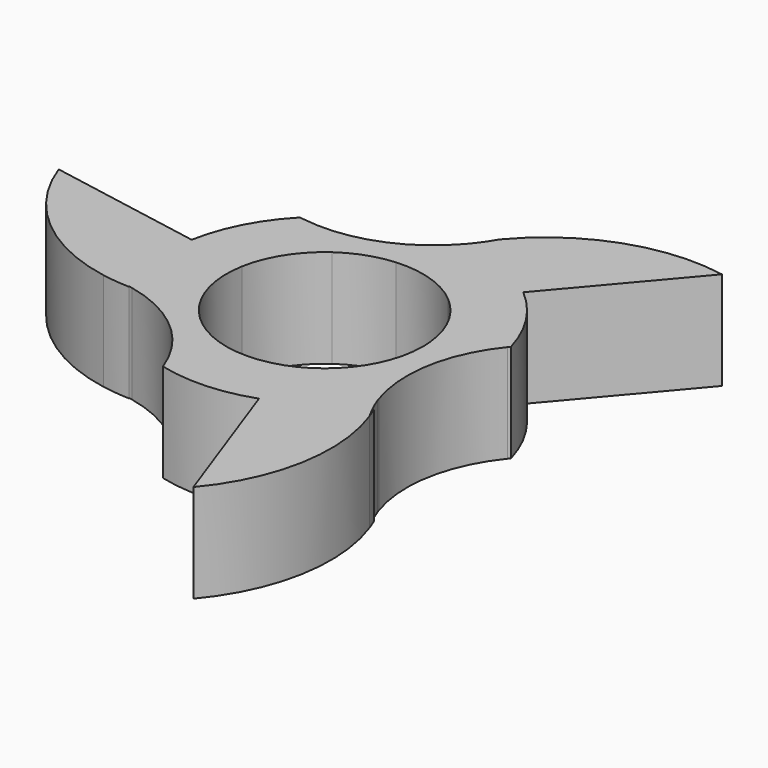
from build123d import *

# Parameters (mm, degrees)
F1_DEPTH = 12.7


# Not quite as in the source:
# - a feature of the source that left no trace in its solid (it failed there, or was rolled back) is left out


with BuildPart() as f1:
    # F0 (on Top) → F1 (new body)
    with BuildSketch(Plane.XY):
        with BuildLine():
            ThreePointArc((-7.3489403011, 10.3577544116), (-4.2883836636, 11.9540689957), (-0.9110245856, 12.667282037))
            ThreePointArc((-0.9110245856, 12.667282037), (0.2194109686, 16.5124994793), (1.9846889119, 20.1107456498))
            ThreePointArc((1.9846889119, 20.1107456498), (-5.3432740228, 15.0903277504), (-14.1828590922, 14.2154720724))
            ThreePointArc((-14.1828590922, 14.2154720724), (-10.6043004202, 12.5728851855), (-7.3489403011, 10.3577544116))
        make_face()
        with BuildLine():
            ThreePointArc((-18.6815829969, -8.250401529), (-18.454845536, -8.2932697378), (-18.2286800533, -8.3390598448))
            ThreePointArc((-18.2286800533, -8.3390598448), (-14.3209728725, -8.0523772846), (-10.5146757481, -7.1226114531))
            ThreePointArc((-10.5146757481, -7.1226114531), (-12.4259555067, -2.6240483505), (-12.4967192607, 2.263185304))
            Line((-12.4967192607, 2.263185304), (-20.0954213497, 3.6393281571))
            ThreePointArc((-20.0954213497, 3.6393281571), (-20.2794337822, -2.4114796562), (-18.6815829969, -8.250401529))
        make_face()
        with BuildLine():
            ThreePointArc((-5.0643582643, -19.7844116422), (0.9578833515, -20.3998315714), (6.8959600381, -19.2228094672))
            Line((6.8959600381, -19.2228094672), (4.2883836636, -11.9540689957))
            ThreePointArc((4.2883836636, -11.9540689957), (-0.5438926438, -12.6883482295), (-5.295608296, -11.5432461975))
            ThreePointArc((-5.295608296, -11.5432461975), (-8.2083355971, -9.6908836917), (-10.5146757481, -7.1226114531))
            ThreePointArc((-10.5146757481, -7.1226114531), (-14.3209728725, -8.0523772846), (-18.2286800533, -8.3390598448))
            ThreePointArc((-18.2286800533, -8.3390598448), (-10.156448241, -12.3478720374), (-5.0643582643, -19.7844116422))
        make_face()
        with BuildLine():
            ThreePointArc((6.8959600381, -19.2228094672), (12.2279291244, -16.3569073478), (16.4855681798, -12.0539085133))
            ThreePointArc((16.4855681798, -12.0539085133), (16.4088993742, -11.8349525851), (16.3350776353, -11.615020425))
            ThreePointArc((16.3350776353, -11.615020425), (14.1333458958, -8.375267358), (11.4257003337, -5.5446705839))
            ThreePointArc((11.4257003337, -5.5446705839), (8.4854702857, -9.4491689598), (4.2883836636, -11.9540689957))
            Line((4.2883836636, -11.9540689957), (6.8959600381, -19.2228094672))
        make_face()
        with BuildLine():
            ThreePointArc((12.6432089432, 1.1996948024), (16.2054891655, 2.9248067913), (19.4293657833, 5.2209930447))
            ThreePointArc((19.4293657833, 5.2209930447), (19.546868725, 5.3645101816), (19.6658540094, 5.5068007715))
            ThreePointArc((19.6658540094, 5.5068007715), (17.187702303, 11.0296671845), (13.1994613117, 15.58348131))
            Line((13.1994613117, 15.58348131), (8.2083355971, 9.6908836917))
            ThreePointArc((8.2083355971, 9.6908836917), (11.2570777566, 5.879472798), (12.6432089432, 1.1996948024))
        make_face()
        with BuildLine():
            ThreePointArc((-0.9110245856, 12.667282037), (3.940485221, 12.0732173104), (8.2083355971, 9.6908836917))
            Line((8.2083355971, 9.6908836917), (13.1994613117, 15.58348131))
            ThreePointArc((13.1994613117, 15.58348131), (8.0325348446, 18.7762896395), (2.1551065289, 20.3082787185))
            ThreePointArc((2.1551065289, 20.3082787185), (2.070257967, 20.2092013887), (1.9846889119, 20.1107456498))
            ThreePointArc((1.9846889119, 20.1107456498), (0.2194109686, 16.5124994793), (-0.9110245856, 12.667282037))
        make_face()
        with BuildLine():
            ThreePointArc((-18.6815829969, -8.250401529), (-20.4319782656, -8.0197287805), (-22.1965884409, -7.9627687686))
            ThreePointArc((-22.1965884409, -7.9627687686), (-20.4281162197, -8.2142893772), (-18.6456789889, -8.3312258223))
            ThreePointArc((-18.6456789889, -8.3312258223), (-18.6636747448, -8.2908331113), (-18.6815829969, -8.250401529))
        make_face()
        with BuildLine():
            ThreePointArc((-40.1908426994, 7.2786563143), (-33.2356793414, -2.7528291756), (-22.1965884409, -7.9627687686))
            Line((-22.1965884409, -7.9627687686), (-40.1908426994, 7.2786563143))
        make_face()
        with BuildLine():
            Line((13.1994613117, 15.58348131), (26.3989226233, 31.1669626201))
            Line((26.3989226233, 31.1669626201), (4.2023341824, 23.2041938515))
            ThreePointArc((4.2023341824, 23.2041938515), (4.1403450601, 23.1307053406), (4.0786560627, 23.0569647133))
            ThreePointArc((4.0786560627, 23.0569647133), (3.1814863156, 21.6374106747), (2.1551065289, 20.3082787185))
            ThreePointArc((2.1551065289, 20.3082787185), (8.0325348446, 18.7762896395), (13.1994613117, 15.58348131))
        make_face()
        with BuildLine():
            Line((4.2023341824, 23.2041938515), (26.3989226233, 31.1669626201))
            ThreePointArc((26.3989226233, 31.1669626201), (14.2338196723, 30.1593572095), (4.2023341824, 23.2041938515))
        make_face()
        with BuildLine():
            ThreePointArc((13.7919200761, -38.4456189344), (19.0018596691, -27.4065280339), (17.9942542585, -15.2414250829))
            Line((17.9942542585, -15.2414250829), (13.7919200761, -38.4456189344))
        make_face()
        with BuildLine():
            ThreePointArc((11.4257003337, -5.5446705839), (14.1333458958, -8.375267358), (16.3350776353, -11.615020425))
            ThreePointArc((16.3350776353, -11.615020425), (15.7367201589, -2.8026923129), (19.4293657833, 5.2209930447))
            ThreePointArc((19.4293657833, 5.2209930447), (16.2054891655, 2.9248067913), (12.6432089432, 1.1996948024))
            ThreePointArc((12.6432089432, 1.1996948024), (12.6857942908, 0.6005191177), (12.7, 0))
            ThreePointArc((12.7, 0), (12.3773259277, -2.8446094426), (11.4257003337, -5.5446705839))
        make_face()
        with BuildLine():
            Line((-20.0954213497, 3.6393281571), (-12.4967192607, 2.263185304))
            ThreePointArc((-12.4967192607, 2.263185304), (-10.7164855769, 6.8151989612), (-7.3489403011, 10.3577544116))
            ThreePointArc((-7.3489403011, 10.3577544116), (-10.6043004202, 12.5728851855), (-14.1828590922, 14.2154720724))
            ThreePointArc((-14.1828590922, 14.2154720724), (-14.3896083966, 14.2484575715), (-14.5959573306, 14.2838614619))
            ThreePointArc((-14.5959573306, 14.2838614619), (-18.1438546347, 9.373964351), (-20.0954213497, 3.6393281571))
        make_face()
        with BuildLine():
            Line((-40.1908426994, 7.2786563143), (-22.1965884409, -7.9627687686))
            ThreePointArc((-22.1965884409, -7.9627687686), (-20.4319782656, -8.0197287805), (-18.6815829969, -8.250401529))
            ThreePointArc((-18.6815829969, -8.250401529), (-20.2794337822, -2.4114796562), (-20.0954213497, 3.6393281571))
            Line((-20.0954213497, 3.6393281571), (-40.1908426994, 7.2786563143))
        make_face()
        with BuildLine():
            Line((13.7919200761, -38.4456189344), (17.9942542585, -15.2414250829))
            ThreePointArc((17.9942542585, -15.2414250829), (17.16114084, -13.6849496708), (16.4855681798, -12.0539085133))
            ThreePointArc((16.4855681798, -12.0539085133), (12.2279291244, -16.3569073478), (6.8959600381, -19.2228094672))
            Line((6.8959600381, -19.2228094672), (13.7919200761, -38.4456189344))
        make_face()
    extrude(amount=F1_DEPTH)


with BuildPart() as f1b:
    # F0 (on Top) → F1, piece 2 (new body)
    with BuildSketch(Plane.XY):
        with BuildLine():
            ThreePointArc((17.4478455198, -13.8573257269), (17.7088929014, -14.5541746878), (17.9942542585, -15.2414250829))
            ThreePointArc((17.9942542585, -15.2414250829), (17.7319700442, -14.5450643934), (17.4478455198, -13.8573257269))
        make_face()
    extrude(amount=F1_DEPTH)


solid = Compound([f1.part, f1b.part])
